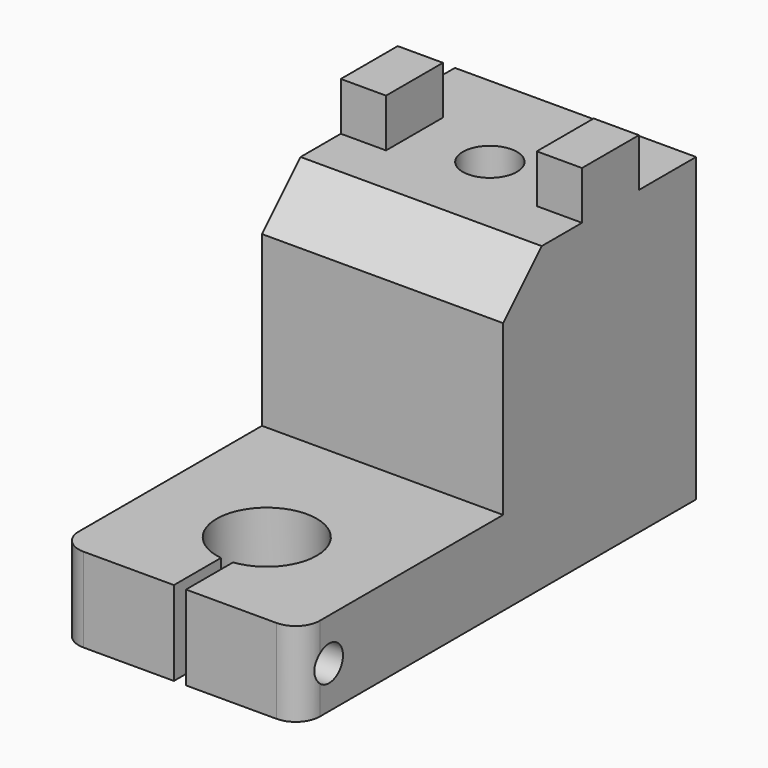
from build123d import *

# Parameters (mm, degrees)
F1_DEPTH    = 7
F2_R        = 1.45
F3_DEPTH    = 25
F4_T1_DEPTH = 17
F5_DEPTH    = 25
F0_W        = 3.75
F0_H        = 5.9
F6_DEPTH    = 29
F7_SIZE     = 4


# Not quite as in the source:
# - a fillet or chamfer that OpenCascade refuses, or shapes differently, is made with other operations: its cross-section is extruded or revolved along the edge and cut away or added
# - a feature names something its author has since deleted; it is built from what else it names


with BuildPart() as f1:
    # F0 (on Top) → F1 (new body)
    with BuildSketch(Plane.XY):
        Polygon((-6.5963959517, 29.175), (-6.5963959517, 21), (13.4036040483, 21), (13.4036040483, 29.175), (9.6536040483, 29.175), (9.6536040483, 35.075), (13.4036040483, 35.075), (13.4036040483, 41), (-6.5963959517, 41), (-6.5963959517, 35.075), (-2.8463959517, 35.075), (-2.8463959517, 29.175), align=None)
        with BuildLine():
            ThreePointArc((1.1536040483, 32.125), (3.4036040483, 34.375), (5.6536040483, 32.125))
            ThreePointArc((5.6536040483, 32.125), (3.4036040483, 29.875), (1.1536040483, 32.125))
        make_face(mode=Mode.SUBTRACT)
        with BuildLine():
            Line((-6.5963959517, 21), (-6.5963959517, 0))
            Line((-6.5963959517, 0), (2.9036040483, 0))
            Line((2.9036040483, 0), (2.9036040483, 4.880230589))
            ThreePointArc((2.9036040483, 4.880230589), (0.6515593539, 12.1062437123), (7.5536040483, 9))
            ThreePointArc((7.5536040483, 9), (6.5098477606, 6.2479553056), (3.9036040483, 4.880230589))
            Line((3.9036040483, 4.880230589), (3.9036040483, 0))
            Line((3.9036040483, 0), (13.4036040483, 0))
            Line((13.4036040483, 0), (13.4036040483, 21))
            Line((13.4036040483, 21), (-6.5963959517, 21))
        make_face()
    extrude(amount=F1_DEPTH)

    # F2 (on face) → F3 (cut)
    with BuildSketch(Plane.YZ.offset(13.4036040483)):
        with Locations((2.95, 3.5)):
            Circle(F2_R)
    extrude(amount=-F3_DEPTH, mode=Mode.SUBTRACT)

    # F4: fillet of radius 2 on 2 edges, made by hand

    # F4_s2 → F4_t1 (cut)
    with BuildSketch(Plane.XY.offset(-5)):
        with BuildLine():
            ThreePointArc((11.4036040483, 0), (12.8178176107, 0.5857864376), (13.4036040483, 2))
            Line((13.4036040483, 2), (13.4036040483, 0))
            Line((13.4036040483, 0), (11.4036040483, 0))
        make_face()
        with BuildLine():
            ThreePointArc((-6.5963959517, 2), (-6.010609514, 0.5857864376), (-4.5963959517, 0))
            Line((-4.5963959517, 0), (-6.5963959517, 0))
            Line((-6.5963959517, 0), (-6.5963959517, 2))
        make_face()
    extrude(amount=F4_T1_DEPTH, mode=Mode.SUBTRACT)

    # F0 (on Top) → F5 (join)
    with BuildSketch(Plane.XY):
        Polygon((-6.5963959517, 29.175), (-6.5963959517, 21), (13.4036040483, 21), (13.4036040483, 29.175), (9.6536040483, 29.175), (9.6536040483, 35.075), (13.4036040483, 35.075), (13.4036040483, 41), (-6.5963959517, 41), (-6.5963959517, 35.075), (-2.8463959517, 35.075), (-2.8463959517, 29.175), align=None)
        with BuildLine():
            ThreePointArc((1.1536040483, 32.125), (3.4036040483, 34.375), (5.6536040483, 32.125))
            ThreePointArc((5.6536040483, 32.125), (3.4036040483, 29.875), (1.1536040483, 32.125))
        make_face(mode=Mode.SUBTRACT)
    extrude(amount=F5_DEPTH)

    # F0 (on Top) → F6 (join)
    with BuildSketch(Plane.XY):
        with Locations((-4.7213959517, 32.125)):
            Rectangle(F0_W, F0_H)
        with Locations((11.5286040483, 32.125)):
            Rectangle(F0_W, F0_H)
    extrude(amount=F6_DEPTH)

    # F7
    f7_edges = [f1.edges().sort_by_distance(p)[0] for p in [
        (3.403604, 21, 25),
    ]]
    chamfer(f7_edges, length=F7_SIZE)


solid = f1.part
